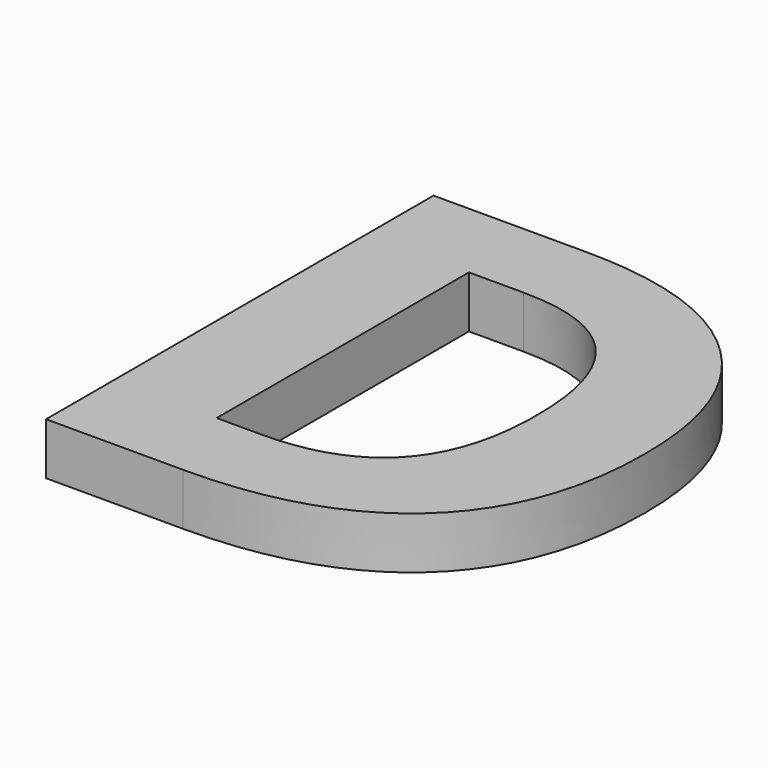
from build123d import *

# Parameters (mm, degrees)
F0_TEXT_SIZE = 66.3224245525
F1_DEPTH     = 5.08


# Not quite as in the source:
# - Text() gives the source's letters only with a copy of the font that has no kerning and outlines rounded to 1/6400 em; it was checked with that copy


with BuildPart() as f1:
    # F0 (on Top) → F1 (new body)
    with BuildSketch(Plane.XY):
        with Locations((0, 0)):
            Text('D', F0_TEXT_SIZE, font='Open Sans', font_style=FontStyle.BOLD, text_align=(TextAlign.LEFT, TextAlign.BOTTOM))
    extrude(amount=F1_DEPTH)


solid = f1.part
